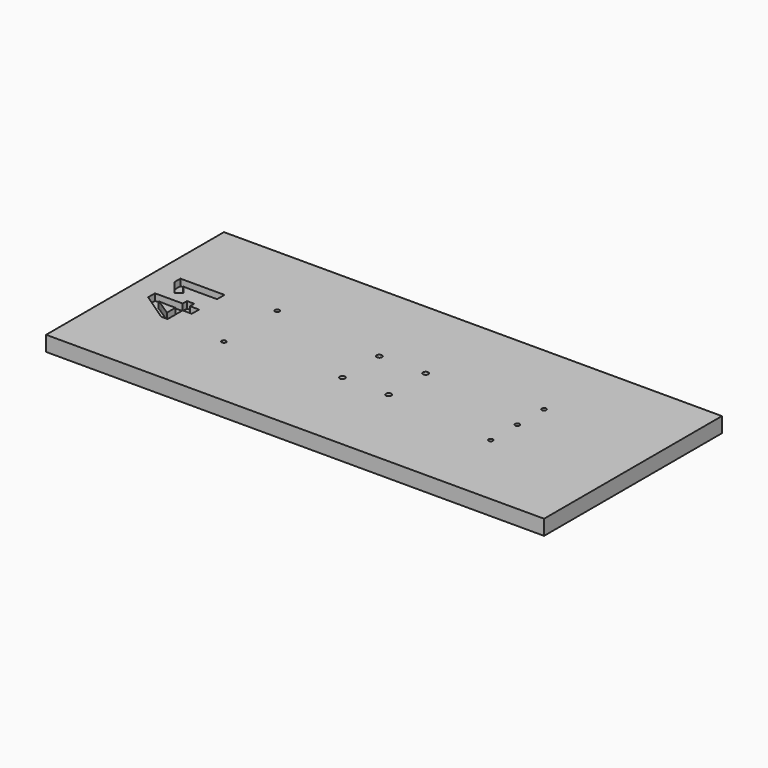
from build123d import *

# Parameters (mm, degrees)
F0_W         = 112
F0_H         = 50
F1_DEPTH     = 3.4
F2_TEXT_SIZE = 13.8888888889
F3_DEPTH     = 1.5
F4_R         = 0.5
F4_R_2       = 0.6
F5_DEPTH     = 3.4


# Not quite as in the source:
# - Text() gives the source's letters only with a copy of the font that has no kerning and outlines rounded to 1/6400 em; it was checked with that copy


with BuildPart() as f1:
    # F0 (on Top) → F1 (new body)
    with BuildSketch(Plane.XY):
        with Locations((12.8412768841, 3.3350909071)):
            Rectangle(F0_W, F0_H)
    extrude(amount=F1_DEPTH)

    # F2 (on face) → F3 (cut)
    with BuildSketch(Plane.XY.offset(3.4)):
        with Locations(Location((-28.1587231159, -3.9149090929), (0, 0, 90))):
            Text('41', F2_TEXT_SIZE, font='Open Sans', font_style=FontStyle.BOLD, text_align=(TextAlign.LEFT, TextAlign.BOTTOM))
    extrude(amount=-F3_DEPTH, mode=Mode.SUBTRACT)

    # F4 (on face) → F5 (cut, through all)
    with BuildSketch(Plane.XY.offset(3.4)):
        with Locations((-17.1587231159, 10.8350909071)):
            Circle(F4_R)
        with Locations((-17.1587231159, -4.1649090929)):
            Circle(F4_R)
        with Locations((7.6412768841, 8.5350909071)):
            Circle(F4_R_2)
        with Locations((18.0412768841, 8.5350909071)):
            Circle(F4_R_2)
        with Locations((18.0412768841, -1.8649090929)):
            Circle(F4_R_2)
        with Locations((7.6412768841, -1.8649090929)):
            Circle(F4_R_2)
        with Locations((42.8412768841, 10.8350909071)):
            Circle(F4_R)
        with Locations((42.8412768841, 3.3350909071)):
            Circle(F4_R)
        with Locations((42.8412768841, -4.1649090929)):
            Circle(F4_R)
    extrude(amount=-F5_DEPTH, mode=Mode.SUBTRACT)


solid = f1.part
